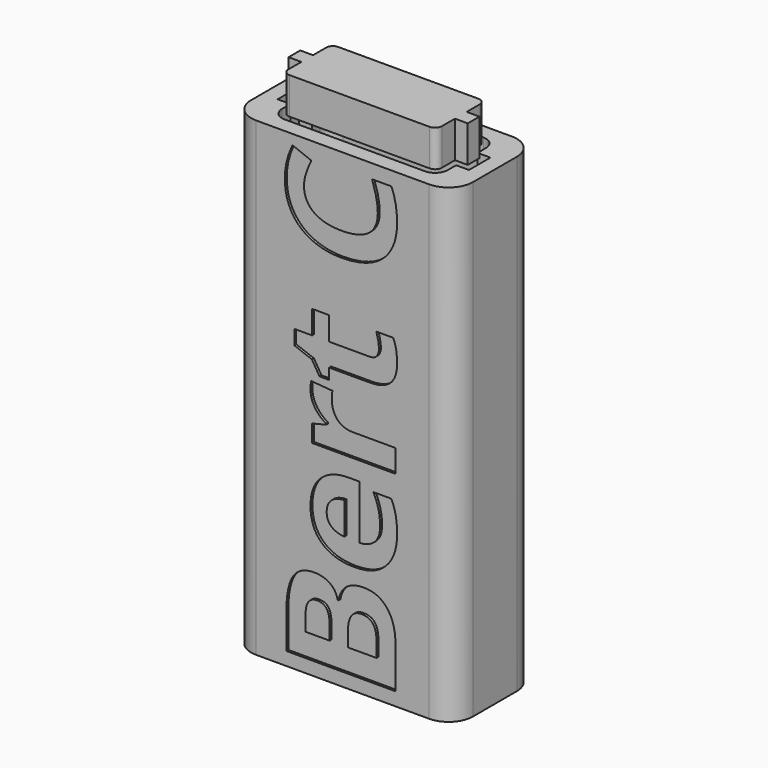
from build123d import *

# Parameters (mm, degrees)
F1_DEPTH     = 36.6
F0_W         = 0.7
F0_H         = 0.3
F0_W_2       = 0.25
F2_DEPTH     = 2
F3_TEXT_SIZE = 12.5558303261
F4_DEPTH     = 0.2
F6_DEPTH     = 3


# Not quite as in the source:
# - Text() gives the source's letters only with a copy of the font that has no kerning and outlines rounded to 1/6400 em; it was checked with that copy


with BuildPart() as f1:
    # F0 (on Top) → F1 (new body)
    with BuildSketch(Plane.XY):
        with BuildLine():
            ThreePointArc((-9.1, -2.35), (-8.5142135624, -3.7642135624), (-7.1, -4.35))
            Line((-7.1, -4.35), (7.1, -4.35))
            ThreePointArc((7.1, -4.35), (8.5142135624, -3.7642135624), (9.1, -2.35))
            Line((9.1, -2.35), (9.1, 2.15))
            ThreePointArc((9.1, 2.15), (8.5142135624, 3.5642135624), (7.1, 4.15))
            Line((7.1, 4.15), (-7.1, 4.15))
            ThreePointArc((-7.1, 4.15), (-8.5142135624, 3.5642135624), (-9.1, 2.15))
            Line((-9.1, 2.15), (-9.1, -2.35))
        make_face()
        with BuildLine():
            Line((-7.85, 1), (-6.8, 1))
            Line((-6.8, 1), (-6.8, 1.85))
            ThreePointArc((-6.8, 1.85), (-6.4924621202, 2.5924621202), (-5.75, 2.9))
            Line((-5.75, 2.9), (5.75, 2.9))
            ThreePointArc((5.75, 2.9), (6.4924621202, 2.5924621202), (6.8, 1.85))
            Line((6.8, 1.85), (6.8, 1))
            Line((6.8, 1), (7.85, 1))
            Line((7.85, 1), (7.85, 0))
            Line((7.85, 0), (7.85, -1.2))
            Line((7.85, -1.2), (6.8, -1.2))
            Line((6.8, -1.2), (6.8, -2.05))
            ThreePointArc((6.8, -2.05), (6.4924621202, -2.7924621202), (5.75, -3.1))
            Line((5.75, -3.1), (-5.75, -3.1))
            ThreePointArc((-5.75, -3.1), (-6.4924621202, -2.7924621202), (-6.8, -2.05))
            Line((-6.8, -2.05), (-6.8, -1.2))
            Line((-6.8, -1.2), (-7.85, -1.2))
            Line((-7.85, -1.2), (-7.85, 0))
            Line((-7.85, 0), (-7.85, 1))
        make_face(mode=Mode.SUBTRACT)
    extrude(amount=F1_DEPTH)

    # F0 (on Top) → F2 (join)
    with BuildSketch(Plane.XY):
        with BuildLine():
            ThreePointArc((-9.1, -2.35), (-8.5142135624, -3.7642135624), (-7.1, -4.35))
            Line((-7.1, -4.35), (7.1, -4.35))
            ThreePointArc((7.1, -4.35), (8.5142135624, -3.7642135624), (9.1, -2.35))
            Line((9.1, -2.35), (9.1, 2.15))
            ThreePointArc((9.1, 2.15), (8.5142135624, 3.5642135624), (7.1, 4.15))
            Line((7.1, 4.15), (-7.1, 4.15))
            ThreePointArc((-7.1, 4.15), (-8.5142135624, 3.5642135624), (-9.1, 2.15))
            Line((-9.1, 2.15), (-9.1, -2.35))
        make_face()
        with BuildLine():
            Line((-7.85, 1), (-6.8, 1))
            Line((-6.8, 1), (-6.8, 1.85))
            ThreePointArc((-6.8, 1.85), (-6.4924621202, 2.5924621202), (-5.75, 2.9))
            Line((-5.75, 2.9), (5.75, 2.9))
            ThreePointArc((5.75, 2.9), (6.4924621202, 2.5924621202), (6.8, 1.85))
            Line((6.8, 1.85), (6.8, 1))
            Line((6.8, 1), (7.85, 1))
            Line((7.85, 1), (7.85, 0))
            Line((7.85, 0), (7.85, -1.2))
            Line((7.85, -1.2), (6.8, -1.2))
            Line((6.8, -1.2), (6.8, -2.05))
            ThreePointArc((6.8, -2.05), (6.4924621202, -2.7924621202), (5.75, -3.1))
            Line((5.75, -3.1), (-5.75, -3.1))
            ThreePointArc((-5.75, -3.1), (-6.4924621202, -2.7924621202), (-6.8, -2.05))
            Line((-6.8, -2.05), (-6.8, -1.2))
            Line((-6.8, -1.2), (-7.85, -1.2))
            Line((-7.85, -1.2), (-7.85, 0))
            Line((-7.85, 0), (-7.85, 1))
        make_face(mode=Mode.SUBTRACT)
        with BuildLine():
            Line((-6.1, -2.05), (-6.1, -0.4))
            Line((-6.1, -0.4), (-6.8, -0.4))
            Line((-6.8, -0.4), (-6.8, -1.2))
            Line((-6.8, -1.2), (-6.8, -2.05))
            ThreePointArc((-6.8, -2.05), (-6.4924621202, -2.7924621202), (-5.75, -3.1))
            Line((-5.75, -3.1), (5.75, -3.1))
            ThreePointArc((5.75, -3.1), (6.4924621202, -2.7924621202), (6.8, -2.05))
            Line((6.8, -2.05), (6.8, -1.2))
            Line((6.8, -1.2), (6.8, -0.4))
            Line((6.8, -0.4), (6.1, -0.4))
            Line((6.1, -0.4), (6.1, -2.05))
            ThreePointArc((6.1, -2.05), (5.9974873734, -2.2974873734), (5.75, -2.4))
            Line((5.75, -2.4), (-5.75, -2.4))
            ThreePointArc((-5.75, -2.4), (-5.9974873734, -2.2974873734), (-6.1, -2.05))
        make_face()
        with BuildLine():
            Line((-6.8, 0.2), (-6.1, 0.2))
            Line((-6.1, 0.2), (-6.1, 0.4))
            Line((-6.1, 0.4), (-6.1, 1.85))
            ThreePointArc((-6.1, 1.85), (-5.9974873734, 2.0974873734), (-5.75, 2.2))
            Line((-5.75, 2.2), (5.75, 2.2))
            ThreePointArc((5.75, 2.2), (5.9974873734, 2.0974873734), (6.1, 1.85))
            Line((6.1, 1.85), (6.1, 0.4))
            Line((6.1, 0.4), (6.1, 0.2))
            Line((6.1, 0.2), (6.8, 0.2))
            Line((6.8, 0.2), (6.8, 1))
            Line((6.8, 1), (6.8, 1.85))
            ThreePointArc((6.8, 1.85), (6.4924621202, 2.5924621202), (5.75, 2.9))
            Line((5.75, 2.9), (-5.75, 2.9))
            ThreePointArc((-5.75, 2.9), (-6.4924621202, 2.5924621202), (-6.8, 1.85))
            Line((-6.8, 1.85), (-6.8, 1))
            Line((-6.8, 1), (-6.8, 0.2))
        make_face()
        Polygon((-7.05, 0.2), (-6.8, 0.2), (-6.8, 1), (-7.85, 1), (-7.85, 0), (-7.85, -1.2), (-6.8, -1.2), (-6.8, -0.4), (-7.05, -0.4), (-7.05, -0.1), align=None)
        Polygon((6.8, 1), (6.8, 0.2), (7.05, 0.2), (7.05, -0.1), (7.05, -0.4), (6.8, -0.4), (6.8, -1.2), (7.85, -1.2), (7.85, 0), (7.85, 1), align=None)
        with Locations((-6.45, -0.25)):
            Rectangle(F0_W, F0_H)
        with Locations((-6.45, 0.05)):
            Rectangle(F0_W, F0_H)
        with Locations((6.45, 0.05)):
            Rectangle(F0_W, F0_H)
        with Locations((6.45, -0.25)):
            Rectangle(F0_W, F0_H)
        with Locations((-6.925, 0.05)):
            Rectangle(F0_W_2, F0_H)
        with Locations((-6.925, -0.25)):
            Rectangle(F0_W_2, F0_H)
        with Locations((6.925, 0.05)):
            Rectangle(F0_W_2, F0_H)
        with Locations((6.925, -0.25)):
            Rectangle(F0_W_2, F0_H)
    extrude(amount=-F2_DEPTH)

    # F3 (on face) → F4 (cut)
    with BuildSketch(Plane.XZ.offset(4.35)):
        with Locations(Location((4.351223477, -2.0405678286), (0, 0, 90))):
            Text('Bert C', F3_TEXT_SIZE, font='Open Sans', font_style=FontStyle.BOLD, text_align=(TextAlign.LEFT, TextAlign.BOTTOM))
    extrude(amount=-F4_DEPTH, mode=Mode.SUBTRACT)


with BuildPart() as f6:
    # F5 (on face) → F6 (new body)
    with BuildSketch(Plane.XY.offset(36.6)):
        with BuildLine():
            Line((6.3, -0.7), (7.35, -0.7))
            Line((7.35, -0.7), (7.35, 0.5))
            Line((7.35, 0.5), (6.3, 0.5))
            Line((6.3, 0.5), (6.3, 1.85))
            ThreePointArc((6.3, 1.85), (6.1389087297, 2.2389087297), (5.75, 2.4))
            Line((5.75, 2.4), (-5.75, 2.4))
            ThreePointArc((-5.75, 2.4), (-6.1389087297, 2.2389087297), (-6.3, 1.85))
            Line((-6.3, 1.85), (-6.3, 0.5))
            Line((-6.3, 0.5), (-7.35, 0.5))
            Line((-7.35, 0.5), (-7.35, -0.7))
            Line((-7.35, -0.7), (-6.3, -0.7))
            Line((-6.3, -0.7), (-6.3, -2.05))
            ThreePointArc((-6.3, -2.05), (-6.1389087297, -2.4389087297), (-5.75, -2.6))
            Line((-5.75, -2.6), (5.75, -2.6))
            ThreePointArc((5.75, -2.6), (6.1389087297, -2.4389087297), (6.3, -2.05))
            Line((6.3, -2.05), (6.3, -0.7))
        make_face()
    extrude(amount=F6_DEPTH)


solid = Compound([f1.part, f6.part])
